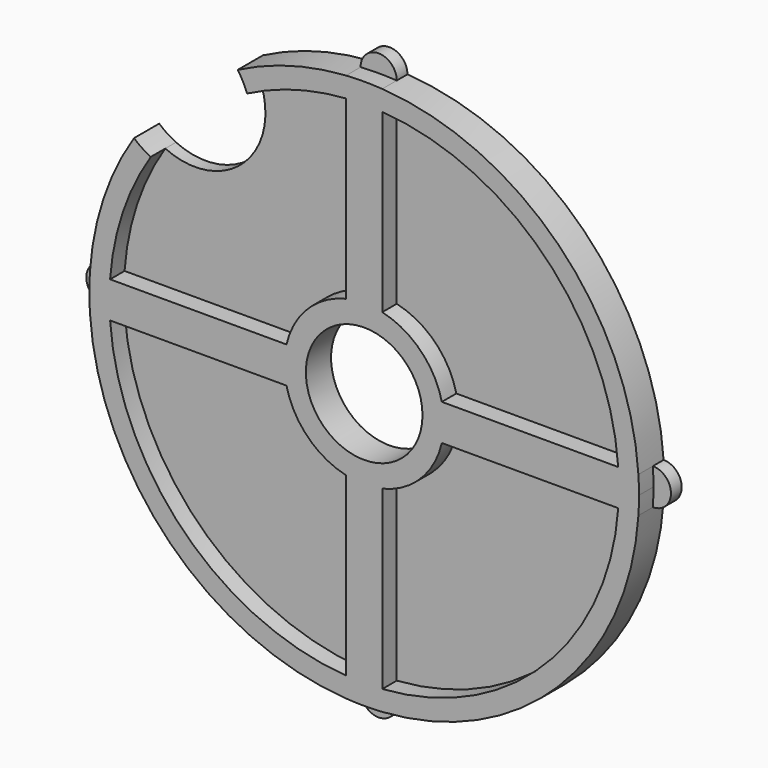
from build123d import *

# Parameters (mm, degrees)
F0_R     = 4.35
F1_DEPTH = 2.35
F2_DEPTH = 1
F3_DEPTH = 25


# Not quite as in the source:
# - a feature names something its author has since deleted; it is built from what else it names


with BuildPart() as f1:
    # F0 (on Front) → F1 (new body)
    with BuildSketch(Plane.XZ):
        with BuildLine():
            ThreePointArc((18.9519787885, 1.35), (18.9879909019, 0.6754269088), (19, 0))
            ThreePointArc((19, 0), (18.9879909019, -0.6754269088), (18.9519787885, -1.35))
            ThreePointArc((18.9519787885, -1.35), (13.4350288425, -13.4350288425), (1.35, -18.9519787885))
            ThreePointArc((1.35, -18.9519787885), (0, -19), (-1.35, -18.9519787885))
            ThreePointArc((-1.35, -18.9519787885), (-13.4350288425, -13.4350288425), (-18.9519787885, -1.35))
            ThreePointArc((-18.9519787885, -1.35), (-19, 0), (-18.9519787885, 1.35))
            ThreePointArc((-18.9519787885, 1.35), (-18.0084373125, 6.0577376603), (-15.9148967645, 10.378634832))
            ThreePointArc((-15.9148967645, 10.378634832), (-16.5717114004, 10.7446905008), (-17.1694954771, 11.2008225173))
            ThreePointArc((-17.1694954771, 11.2008225173), (-19.4465872664, 6.4869286792), (-20.4555004828, 1.35))
            ThreePointArc((-20.4555004828, 1.35), (-20.5, 0), (-20.4555004828, -1.35))
            ThreePointArc((-20.4555004828, -1.35), (-14.4956890143, -14.4956890143), (-1.35, -20.4555004828))
            ThreePointArc((-1.35, -20.4555004828), (0, -20.5), (1.35, -20.4555004828))
            ThreePointArc((1.35, -20.4555004828), (14.4956890143, -14.4956890143), (20.4555004828, -1.35))
            ThreePointArc((20.4555004828, -1.35), (20.4888721004, -0.6753666055), (20.5, 0))
            ThreePointArc((20.5, 0), (20.4888721004, 0.6753666055), (20.4555004828, 1.35))
            ThreePointArc((20.4555004828, 1.35), (14.4956890143, 14.4956890143), (1.35, 20.4555004828))
            ThreePointArc((1.35, 20.4555004828), (0, 20.5), (-1.35, 20.4555004828))
            ThreePointArc((-1.35, 20.4555004828), (-5.5075668443, 19.7463087046), (-9.4320097524, 18.2012964382))
            ThreePointArc((-9.4320097524, 18.2012964382), (-9.0377919084, 17.5609883013), (-8.7390902551, 16.8709306653))
            ThreePointArc((-8.7390902551, 16.8709306653), (-5.1507403222, 18.2885175488), (-1.35, 18.9519787885))
            ThreePointArc((-1.35, 18.9519787885), (0, 19), (1.35, 18.9519787885))
            ThreePointArc((1.35, 18.9519787885), (13.4350288425, 13.4350288425), (18.9519787885, 1.35))
        make_face()
        with BuildLine():
            ThreePointArc((-1.35, -18.9519787885), (0, -19), (1.35, -18.9519787885))
            Line((1.35, -18.9519787885), (1.35, -5.7948252778))
            ThreePointArc((1.35, -5.7948252778), (0, -5.95), (-1.35, -5.7948252778))
            Line((-1.35, -5.7948252778), (-1.35, -18.9519787885))
        make_face()
        with BuildLine():
            ThreePointArc((18.9519787885, -1.35), (18.9879909019, -0.6754269088), (19, 0))
            ThreePointArc((19, 0), (18.9879909019, 0.6754269088), (18.9519787885, 1.35))
            Line((18.9519787885, 1.35), (5.7948252778, 1.35))
            ThreePointArc((5.7948252778, 1.35), (5.9110790218, 0.6794444779), (5.95, 0))
            ThreePointArc((5.95, 0), (5.9110790218, -0.6794444779), (5.7948252778, -1.35))
            Line((5.7948252778, -1.35), (18.9519787885, -1.35))
        make_face()
        with BuildLine():
            ThreePointArc((-18.9519787885, 1.35), (-19, 0), (-18.9519787885, -1.35))
            Line((-18.9519787885, -1.35), (-5.7948252778, -1.35))
            ThreePointArc((-5.7948252778, -1.35), (-5.95, 0), (-5.7948252778, 1.35))
            Line((-5.7948252778, 1.35), (-18.9519787885, 1.35))
        make_face()
        with BuildLine():
            Line((1.35, 5.7948252778), (1.35, 18.9519787885))
            ThreePointArc((1.35, 18.9519787885), (0, 19), (-1.35, 18.9519787885))
            Line((-1.35, 18.9519787885), (-1.35, 5.7948252778))
            ThreePointArc((-1.35, 5.7948252778), (0, 5.95), (1.35, 5.7948252778))
        make_face()
        with BuildLine():
            ThreePointArc((5.95, 0), (5.9110790218, 0.6794444779), (5.7948252778, 1.35))
            ThreePointArc((5.7948252778, 1.35), (4.2072853481, 4.2072853481), (1.35, 5.7948252778))
            ThreePointArc((1.35, 5.7948252778), (0, 5.95), (-1.35, 5.7948252778))
            ThreePointArc((-1.35, 5.7948252778), (-4.2072853481, 4.2072853481), (-5.7948252778, 1.35))
            ThreePointArc((-5.7948252778, 1.35), (-5.95, 0), (-5.7948252778, -1.35))
            ThreePointArc((-5.7948252778, -1.35), (-4.2072853481, -4.2072853481), (-1.35, -5.7948252778))
            ThreePointArc((-1.35, -5.7948252778), (0, -5.95), (1.35, -5.7948252778))
            ThreePointArc((1.35, -5.7948252778), (4.2072853481, -4.2072853481), (5.7948252778, -1.35))
            ThreePointArc((5.7948252778, -1.35), (5.9110790218, -0.6794444779), (5.95, 0))
        make_face()
        Circle(F0_R, mode=Mode.SUBTRACT)
    extrude(amount=F1_DEPTH)

    # F0 (on Front) → F2 (join)
    with BuildSketch(Plane.XZ):
        with BuildLine():
            Line((-1.35, 5.7948252778), (-1.35, 18.9519787885))
            ThreePointArc((-1.35, 18.9519787885), (-5.1507403222, 18.2885175488), (-8.7390902551, 16.8709306653))
            ThreePointArc((-8.7390902551, 16.8709306653), (-10.1717962693, 11.2426857548), (-15.9148967645, 10.378634832))
            ThreePointArc((-15.9148967645, 10.378634832), (-18.0084373125, 6.0577376603), (-18.9519787885, 1.35))
            Line((-18.9519787885, 1.35), (-5.7948252778, 1.35))
            ThreePointArc((-5.7948252778, 1.35), (-4.2072853481, 4.2072853481), (-1.35, 5.7948252778))
        make_face()
        with BuildLine():
            ThreePointArc((1.35, -18.9519787885), (13.4350288425, -13.4350288425), (18.9519787885, -1.35))
            Line((18.9519787885, -1.35), (5.7948252778, -1.35))
            ThreePointArc((5.7948252778, -1.35), (4.2072853481, -4.2072853481), (1.35, -5.7948252778))
            Line((1.35, -5.7948252778), (1.35, -18.9519787885))
        make_face()
        with BuildLine():
            Line((5.7948252778, 1.35), (18.9519787885, 1.35))
            ThreePointArc((18.9519787885, 1.35), (13.4350288425, 13.4350288425), (1.35, 18.9519787885))
            Line((1.35, 18.9519787885), (1.35, 5.7948252778))
            ThreePointArc((1.35, 5.7948252778), (4.2072853481, 4.2072853481), (5.7948252778, 1.35))
        make_face()
        with BuildLine():
            ThreePointArc((-18.9519787885, -1.35), (-13.4350288425, -13.4350288425), (-1.35, -18.9519787885))
            Line((-1.35, -18.9519787885), (-1.35, -5.7948252778))
            ThreePointArc((-1.35, -5.7948252778), (-4.2072853481, -4.2072853481), (-5.7948252778, -1.35))
            Line((-5.7948252778, -1.35), (-18.9519787885, -1.35))
        make_face()
        with BuildLine():
            ThreePointArc((-20.4555004828, -1.35), (-20.5, 0), (-20.4555004828, 1.35))
            ThreePointArc((-20.4555004828, 1.35), (-21.8055004828, 0), (-20.4555004828, -1.35))
        make_face()
        with BuildLine():
            ThreePointArc((1.35, -20.4555004828), (0, -20.5), (-1.35, -20.4555004828))
            ThreePointArc((-1.35, -20.4555004828), (0, -21.8055004828), (1.35, -20.4555004828))
        make_face()
        with BuildLine():
            ThreePointArc((20.4555004828, -1.35), (21.8055004828, 0), (20.4555004828, 1.35))
            ThreePointArc((20.4555004828, 1.35), (20.4888721004, 0.6753666055), (20.5, 0))
            ThreePointArc((20.5, 0), (20.4888721004, -0.6753666055), (20.4555004828, -1.35))
        make_face()
        with BuildLine():
            ThreePointArc((1.35, 20.4555004828), (0, 21.8055004828), (-1.35, 20.4555004828))
            ThreePointArc((-1.35, 20.4555004828), (0, 20.5), (1.35, 20.4555004828))
        make_face()
    extrude(amount=F2_DEPTH)

    # F0 (on Front) → F3 (cut)
    with BuildSketch(Plane.XZ):
        with BuildLine():
            ThreePointArc((18.9519787885, 1.35), (18.9879909019, 0.6754269088), (19, 0))
            ThreePointArc((19, 0), (18.9879909019, -0.6754269088), (18.9519787885, -1.35))
            ThreePointArc((18.9519787885, -1.35), (13.4350288425, -13.4350288425), (1.35, -18.9519787885))
            ThreePointArc((1.35, -18.9519787885), (0, -19), (-1.35, -18.9519787885))
            ThreePointArc((-1.35, -18.9519787885), (-13.4350288425, -13.4350288425), (-18.9519787885, -1.35))
            ThreePointArc((-18.9519787885, -1.35), (-19, 0), (-18.9519787885, 1.35))
            ThreePointArc((-18.9519787885, 1.35), (-18.0084373125, 6.0577376603), (-15.9148967645, 10.378634832))
            ThreePointArc((-15.9148967645, 10.378634832), (-16.5717114004, 10.7446905008), (-17.1694954771, 11.2008225173))
            ThreePointArc((-17.1694954771, 11.2008225173), (-19.4465872664, 6.4869286792), (-20.4555004828, 1.35))
            ThreePointArc((-20.4555004828, 1.35), (-20.5, 0), (-20.4555004828, -1.35))
            ThreePointArc((-20.4555004828, -1.35), (-14.4956890143, -14.4956890143), (-1.35, -20.4555004828))
            ThreePointArc((-1.35, -20.4555004828), (0, -20.5), (1.35, -20.4555004828))
            ThreePointArc((1.35, -20.4555004828), (14.4956890143, -14.4956890143), (20.4555004828, -1.35))
            ThreePointArc((20.4555004828, -1.35), (20.4888721004, -0.6753666055), (20.5, 0))
            ThreePointArc((20.5, 0), (20.4888721004, 0.6753666055), (20.4555004828, 1.35))
            ThreePointArc((20.4555004828, 1.35), (14.4956890143, 14.4956890143), (1.35, 20.4555004828))
            ThreePointArc((1.35, 20.4555004828), (0, 20.5), (-1.35, 20.4555004828))
            ThreePointArc((-1.35, 20.4555004828), (-5.5075668443, 19.7463087046), (-9.4320097524, 18.2012964382))
            ThreePointArc((-9.4320097524, 18.2012964382), (-9.0377919084, 17.5609883013), (-8.7390902551, 16.8709306653))
            ThreePointArc((-8.7390902551, 16.8709306653), (-5.1507403222, 18.2885175488), (-1.35, 18.9519787885))
            ThreePointArc((-1.35, 18.9519787885), (0, 19), (1.35, 18.9519787885))
            ThreePointArc((1.35, 18.9519787885), (13.4350288425, 13.4350288425), (18.9519787885, 1.35))
        make_face()
        with BuildLine():
            ThreePointArc((-15.9148967645, 10.378634832), (-12.7472446155, 14.0892780054), (-8.7390902551, 16.8709306653))
            ThreePointArc((-8.7390902551, 16.8709306653), (-9.0377919084, 17.5609883013), (-9.4320097524, 18.2012964382))
            ThreePointArc((-9.4320097524, 18.2012964382), (-13.7536060325, 15.2015894268), (-17.1694954771, 11.2008225173))
            ThreePointArc((-17.1694954771, 11.2008225173), (-16.5717114004, 10.7446905008), (-15.9148967645, 10.378634832))
        make_face()
        with BuildLine():
            ThreePointArc((1.35, 20.4555004828), (0, 21.8055004828), (-1.35, 20.4555004828))
            ThreePointArc((-1.35, 20.4555004828), (0, 20.5), (1.35, 20.4555004828))
        make_face()
        with BuildLine():
            ThreePointArc((-20.4555004828, -1.35), (-20.5, 0), (-20.4555004828, 1.35))
            ThreePointArc((-20.4555004828, 1.35), (-21.8055004828, 0), (-20.4555004828, -1.35))
        make_face()
        with BuildLine():
            ThreePointArc((20.4555004828, -1.35), (21.8055004828, 0), (20.4555004828, 1.35))
            ThreePointArc((20.4555004828, 1.35), (20.4888721004, 0.6753666055), (20.5, 0))
            ThreePointArc((20.5, 0), (20.4888721004, -0.6753666055), (20.4555004828, -1.35))
        make_face()
        with BuildLine():
            ThreePointArc((1.35, -20.4555004828), (0, -20.5), (-1.35, -20.4555004828))
            ThreePointArc((-1.35, -20.4555004828), (0, -21.8055004828), (1.35, -20.4555004828))
        make_face()
    extrude(amount=-F3_DEPTH, mode=Mode.SUBTRACT)


solid = f1.part
